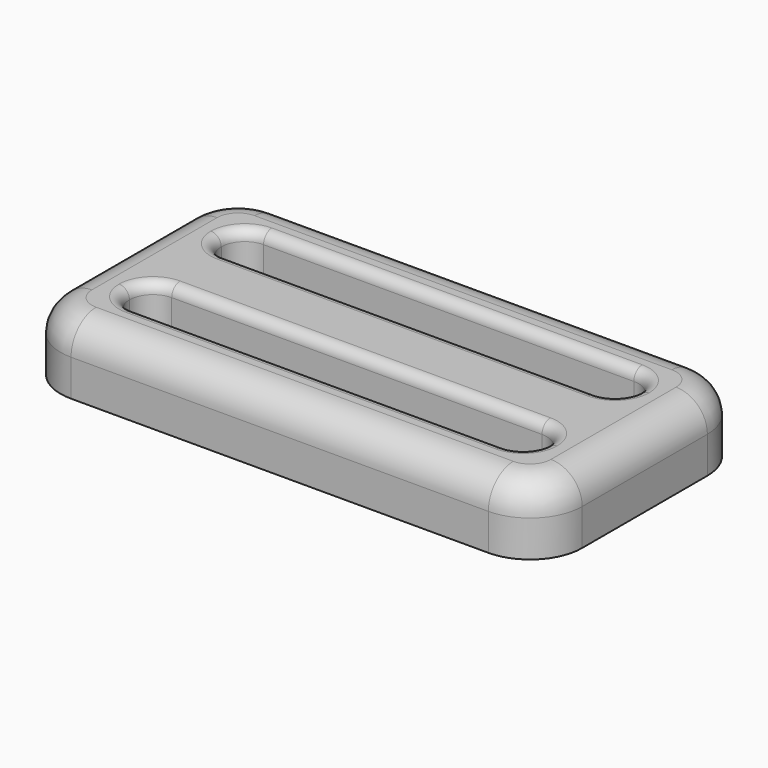
from build123d import *

# Parameters (mm, degrees)
F0_W     = 50
F0_H     = 25
F0_W_2   = 40
F0_H_2   = 4.5
F1_DEPTH = 6.5
F2_R     = 5
F3_R     = 2.24999
F4_R     = 1
F5_R     = 3


# Not quite as in the source:
# - a fillet or chamfer is up to 0.001 mm smaller than in the source, because OpenCascade refuses the exact size


with BuildPart() as f1:
    # F0 (on Top) → F1 (new body)
    with BuildSketch(Plane.XY):
        Rectangle(F0_W, F0_H)
        with Locations((0, -5.5)):
            Rectangle(F0_W_2, F0_H_2, mode=Mode.SUBTRACT)
        with Locations((0, 5.5)):
            Rectangle(F0_W_2, F0_H_2, mode=Mode.SUBTRACT)
    extrude(amount=F1_DEPTH)

    # F2
    f2_edges = [f1.edges().sort_by_distance(p)[0] for p in [
        (-25, -12.5, 3.25),
        (25, -12.5, 3.25),
        (25, 12.5, 3.25),
        (-25, 12.5, 3.25),
    ]]
    fillet(f2_edges, radius=F2_R)

    # F3 (radius 2.25 in the source; OpenCascade refuses exactly that, so slightly less here)
    f3_edges = [f1.edges().sort_by_distance(p)[0] for p in [
        (-20, -3.25, 3.25),
        (-20, -7.75, 3.25),
        (-20, 3.25, 3.25),
        (-20, 7.75, 3.25),
        (20, -7.75, 3.25),
        (20, -3.25, 3.25),
        (20, 3.25, 3.25),
        (20, 7.75, 3.25),
    ]]
    fillet(f3_edges, radius=F3_R)

    # F4
    f4_edges = [f1.edges().sort_by_distance(p)[0] for p in [
        (0, -7.75, 6.5),
        (0, 3.25, 6.5),
    ]]
    fillet(f4_edges, radius=F4_R)

    # F5
    f5_edges = [f1.edges().sort_by_distance(p)[0] for p in [
        (25, 0, 6.5),
    ]]
    fillet(f5_edges, radius=F5_R)


solid = f1.part
